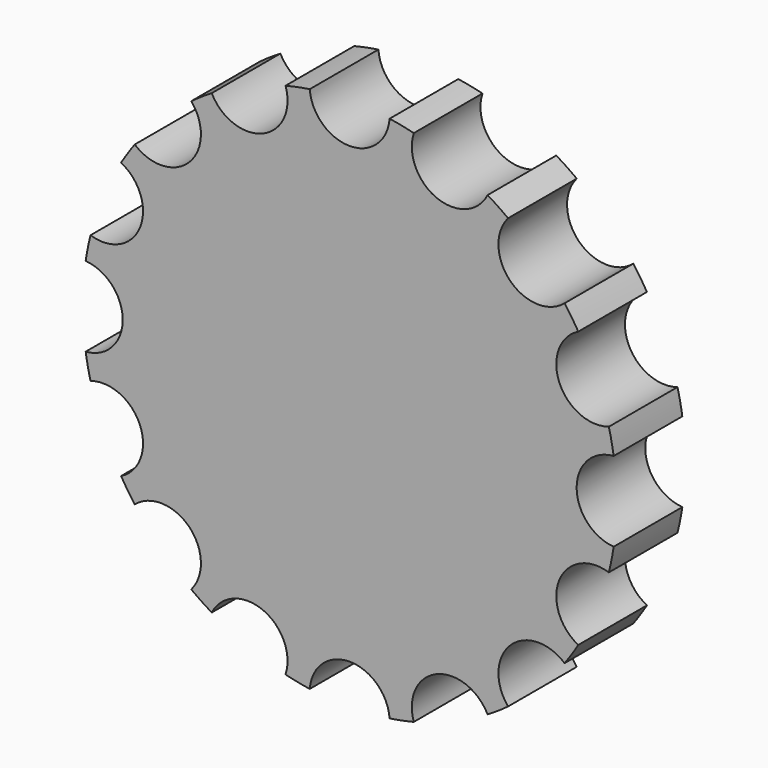
from build123d import *

# Parameters (mm, degrees)
F0_R            = 14
F1_DEPTH        = 4.5
F3_DEPTH        = 4.501
F3_COPIES_COUNT = 16


# Not quite as in the source:
# - a pattern or mirror of a feature is missing from the dataset's text; its kind, count and spacing are read off the source's solid


with BuildPart() as f1:
    # F0 (on Front) → F1 (new body)
    with BuildSketch(Plane.XZ):
        Circle(F0_R)
    extrude(amount=F1_DEPTH)

    # F2 (on face) → F3 (cut, through all)
    with BuildSketch(Plane.XZ.offset(4.5)):
        with BuildLine():
            ThreePointArc((2.0940854209, 13.8425), (0, 14), (-2.0940854209, 13.8425))
            ThreePointArc((-2.0940854209, 13.8425), (0, 11.9), (2.0940854209, 13.8425))
        make_face()
    f3 = extrude(amount=-F3_DEPTH, mode=Mode.SUBTRACT)

    # F3_copies: F3 ×16 about axis
    f3_copies_axis = Axis((0, 0, 0), (0, 1, 0))
    for i in range(1, F3_COPIES_COUNT):
        add(f3.rotate(f3_copies_axis, i * 360 / F3_COPIES_COUNT), mode=Mode.SUBTRACT)


solid = f1.part
